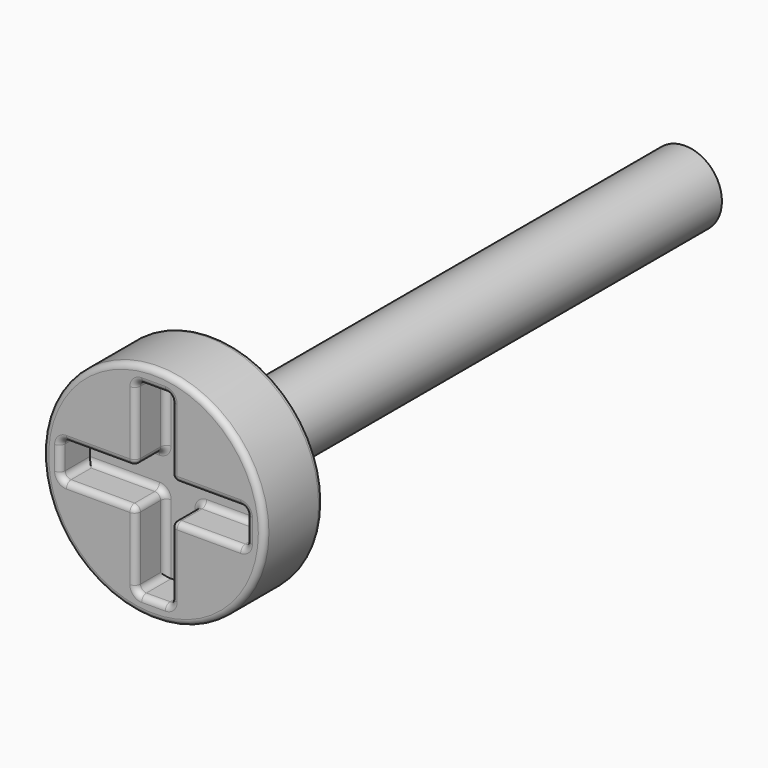
from build123d import *

# Parameters (mm, degrees)
F0_R     = 1.5875
F1_DEPTH = 12.7
F2_R     = 4.7625
F3_DEPTH = 3.175
F4_W     = 1.524
F4_H     = 3.2385
F4_H_2   = 1.524
F4_W_2   = 3.2385
F5_DEPTH = 1.5875
F6_R     = 0.254


with BuildPart() as f1:
    # F0 (on Front) → F1 (new body, symmetric)
    with BuildSketch(Plane.XZ):
        Circle(F0_R)
    extrude(amount=F1_DEPTH, both=True)

    # F2 (on face) → F3 (join)
    with BuildSketch(Plane.XZ.offset(12.7)):
        Circle(F2_R)
    extrude(amount=F3_DEPTH)

    # F4 (on face) → F5 (cut)
    with BuildSketch(Plane.XZ.offset(15.875)):
        with Locations((0, 2.38125)):
            Rectangle(F4_W, F4_H)
        Rectangle(F4_W, F4_H_2)
        with Locations((-2.38125, 0)):
            Rectangle(F4_W_2, F4_H_2)
        with Locations((2.38125, 0)):
            Rectangle(F4_W_2, F4_H_2)
        with Locations((0, -2.38125)):
            Rectangle(F4_W, F4_H)
    extrude(amount=-F5_DEPTH, mode=Mode.SUBTRACT)

    # F6
    f6_edges = [f1.edges().sort_by_distance(p)[0] for p in [
        (-4.7625, -15.875, 0),
        (-2.38125, -15.875, 0.762),
        (-0.762, -15.875, 2.38125),
        (0.762, -15.875, 2.38125),
        (-2.38125, -15.875, -0.762),
        (-0.762, -15.875, -2.38125),
        (2.38125, -15.875, -0.762),
        (2.38125, -15.875, 0.762),
        (-0.762, -15.08125, 0.762),
        (-4.0005, -15.08125, 0.762),
        (-2.38125, -14.2875, 0.762),
        (4.0005, -15.08125, 0.762),
        (0.762, -15.08125, 0.762),
        (2.38125, -14.2875, 0.762),
        (-4.0005, -15.08125, -0.762),
        (-0.762, -15.08125, -0.762),
        (-2.38125, -14.2875, -0.762),
        (0.762, -15.08125, -0.762),
        (4.0005, -15.08125, -0.762),
        (2.38125, -14.2875, -0.762),
        (0, -15.875, 4.0005),
        (0, -15.875, -4.0005),
        (0.762, -15.08125, 4.0005),
        (-0.762, -15.08125, 4.0005),
        (0.762, -15.08125, -4.0005),
        (-0.762, -15.08125, -4.0005),
        (-4.7625, -12.7, 0),
        (-4.0005, -15.875, 0),
        (0.762, -15.875, -2.38125),
        (4.0005, -15.875, 0),
        (-0.762, -14.2875, 2.38125),
        (-0.762, -14.2875, -2.38125),
        (0.762, -14.2875, -2.38125),
        (0.762, -14.2875, 2.38125),
    ]]
    fillet(f6_edges, radius=F6_R)


solid = f1.part
